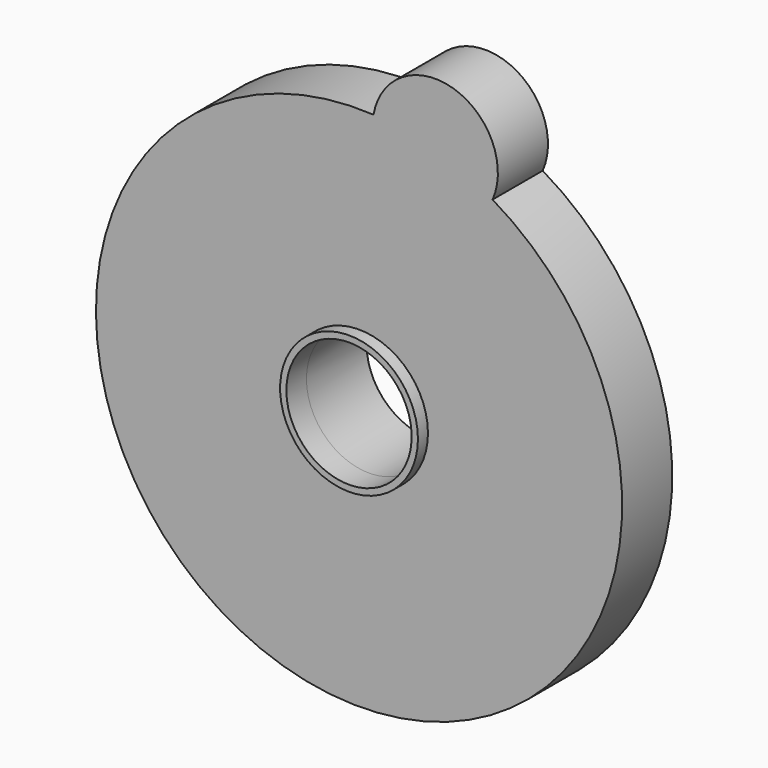
from build123d import *
from build123d import SkipClean  # not in build123d's __all__

# Parameters (mm, degrees)
F2_R      = 21
F3_DEPTH  = 3
F4_R      = 10
F5_DEPTH  = 2
F6_R      = 5
F7_DEPTH  = 25
F8_R      = 5
F9_DEPTH  = 3
F10_R     = 5.5
F11_DEPTH = 1
F12_DEPTH = 1
F13_R     = 5.5
F14_DEPTH = 1
F15_R     = 5
F16_DEPTH = 1
F17_DEPTH = 2


# Not quite as in the source:
# - the program builds the solid bodies; features that only make, move or delete a surface that nothing else refers to are left out


with BuildPart() as f3:
    # F2 (on Front) → F3 (new body)
    with BuildSketch(Plane.XZ):
        Circle(F2_R)
    extrude(amount=F3_DEPTH)

    # F4 (on Front) → F5 (join)
    with BuildSketch(Plane.XZ):
        Circle(F4_R)
    extrude(amount=-F5_DEPTH)

    # F6 (on face) → F7 (cut)
    with BuildSketch(Plane(origin=(0, 2, 0), x_dir=(-1, 0, 0), z_dir=(0, 1, 0))):
        Circle(F6_R)
    extrude(amount=-F7_DEPTH, mode=Mode.SUBTRACT)

    # F8 (on face) → F9 (join)
    with BuildSketch(Plane.XZ.offset(3)):
        with Locations((6.0798030726, 20.1006466214)):
            Circle(F8_R)
        with BuildLine():
            ThreePointArc((10.6593068139, 18.093622585), (6.0798030726, 20.1006466214), (1.1556392931, 20.968178219))
            ThreePointArc((1.1556392931, 20.968178219), (4.6322309124, 15.3147783782), (10.6593068139, 18.093622585))
        make_face()
    extrude(amount=-F9_DEPTH)

    # F10 (on face) → F11 (join)
    with BuildSketch(Plane.XZ.offset(3)):
        with BuildLine():
            ThreePointArc((10.6593068139, 18.093622585), (7.5273752327, 24.8865148646), (1.1556392931, 20.968178219))
            ThreePointArc((1.1556392931, 20.968178219), (-6.0798030726, -20.1006466214), (10.6593068139, 18.093622585))
        make_face()
        Circle(F10_R, mode=Mode.SUBTRACT)
    with SkipClean():  # cleaning this boolean's faces spoils the solid; the shape is the same uncleaned
        extrude(amount=F11_DEPTH)

    # F12 (add): a face of the model
    f12_faces = [f3.faces().sort_by_distance(p)[0] for p in [
        (-5.3444365081, -3, 0),
    ]]
    with SkipClean():  # cleaning this boolean's faces spoils the solid; the shape is the same uncleaned
        extrude(f12_faces, amount=F12_DEPTH)

    # F13 (on face) → F14 (join)
    with BuildSketch(Plane.XZ.offset(4)):
        with BuildLine():
            ThreePointArc((10.6593068139, 18.093622585), (7.5273752327, 24.8865148646), (1.1556392931, 20.968178219))
            ThreePointArc((1.1556392931, 20.968178219), (-6.0798030726, -20.1006466214), (10.6593068139, 18.093622585))
        make_face()
        Circle(F13_R, mode=Mode.SUBTRACT)
    extrude(amount=F14_DEPTH)

    # F15 (on face) → F16 (cut)
    with BuildSketch(Plane.XZ.offset(5)):
        Circle(F15_R)
    extrude(amount=-F16_DEPTH, mode=Mode.SUBTRACT)

    # F17 (add): a face of the model
    f17_faces = [f3.faces().sort_by_distance(p)[0] for p in [
        (-5.3444365081, -4, 0),
    ]]
    extrude(f17_faces, amount=F17_DEPTH)


solid = f3.part
